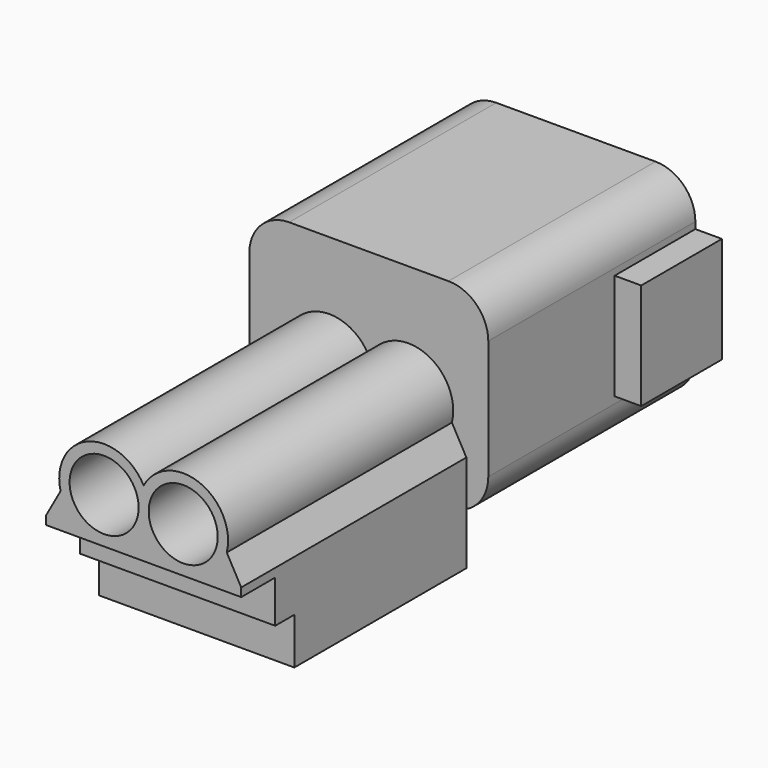
from build123d import *

# Parameters (mm, degrees)
F1_DEPTH     = 21.2
F2_W         = 14.7
F2_H         = 3.2
F3_DEPTH     = 6.7
F4_R         = 2.6
F5_DEPTH     = 10
F6_W         = 18
F6_H         = 15
F7_DEPTH     = 11.9
F9_DEPTH     = 7.6
F10_T1_DEPTH = 34.5
F10_T3_DEPTH = 27
F11_W        = 14.7
F11_H        = 1.8
F12_DEPTH    = 3.5


# Not quite as in the source:
# - a fillet or chamfer that OpenCascade refuses, or shapes differently, is made with other operations: its cross-section is extruded or revolved along the edge and cut away or added


with BuildPart() as f1:
    # F0 (on Front) → F1 (new body)
    with BuildSketch(Plane.XZ):
        with BuildLine():
            Line((-7.35, 0.194197055), (-7.35, -7.15))
            Line((-7.35, -7.15), (7.35, -7.15))
            Line((7.35, -7.15), (7.35, 0.194197055))
            Line((7.35, 0.194197055), (6.2603328375, 2.1552506672))
            ThreePointArc((6.2603328375, 2.1552506672), (3.3980247264, -0.3840505852), (0, 1.375007837))
            ThreePointArc((0, 1.375007837), (-3.3980247264, -0.3840505852), (-6.2603328375, 2.1552506672))
            Line((-6.2603328375, 2.1552506672), (-7.35, 0.194197055))
        make_face()
        with BuildLine():
            ThreePointArc((0, 4.564992163), (-4.1941925187, 6.1243837001), (-6.2603328375, 2.1552506672))
            ThreePointArc((-6.2603328375, 2.1552506672), (-3.3980247264, -0.3840505852), (0, 1.375007837))
            ThreePointArc((0, 1.375007837), (3.3980247264, -0.3840505852), (6.2603328375, 2.1552506672))
            ThreePointArc((6.2603328375, 2.1552506672), (4.1941925187, 6.1243837001), (0, 4.564992163))
        make_face()
    extrude(amount=F1_DEPTH)

    # F2 (on face) → F3 (cut)
    with BuildSketch(Plane(origin=(0, 0, -7.15), x_dir=(1, 0, 0), z_dir=(0, 0, -1))):
        with Locations((0, 19.6)):
            Rectangle(F2_W, F2_H)
    extrude(amount=-F3_DEPTH, mode=Mode.SUBTRACT)

    # F4 (on face) → F5 (cut)
    with BuildSketch(Plane.XZ.offset(21.2)):
        with Locations((-2.98, 2.97)):
            Circle(F4_R)
        with Locations((2.98, 2.97)):
            Circle(F4_R)
    extrude(amount=-F5_DEPTH, mode=Mode.SUBTRACT)

    # F6 (on face) → F7 (join)
    with BuildSketch(Plane(origin=(0, 0, 0), x_dir=(-1, 0, 0), z_dir=(0, 1, 0))):
        with Locations((0, 3.95)):
            Rectangle(F6_W, F6_H)
    extrude(amount=F7_DEPTH)

    # F8 (on face) → F9 (join)
    with BuildSketch(Plane(origin=(0, 11.9, 0), x_dir=(-1, 0, 0), z_dir=(0, 1, 0))):
        Polygon((-9, -0.05), (-9, -3.55), (9, -3.55), (9, -0.05), (11, -0.05), (11, 7.95), (9, 7.95), (9, 11.45), (-9, 11.45), (-9, 7.95), (-11, 7.95), (-11, -0.05), align=None)
    extrude(amount=F9_DEPTH)

    # F10: fillet of radius 3 on 4 edges, made by hand

    # F10_s2 → F10_t1 (cut)
    with BuildSketch(Plane.XZ.offset(-27)):
        with BuildLine():
            ThreePointArc((6, 11.45), (8.1213203436, 10.5713203436), (9, 8.45))
            Line((9, 8.45), (9, 11.45))
            Line((9, 11.45), (6, 11.45))
        make_face()
        with BuildLine():
            ThreePointArc((-9, 8.45), (-8.1213203436, 10.5713203436), (-6, 11.45))
            Line((-6, 11.45), (-9, 11.45))
            Line((-9, 11.45), (-9, 8.45))
        make_face()
    extrude(amount=F10_T1_DEPTH, mode=Mode.SUBTRACT)

    # F10_s4 → F10_t3 (cut)
    with BuildSketch(Plane.XZ.offset(-27)):
        with BuildLine():
            ThreePointArc((6, -3.55), (8.1213203436, -2.6713203436), (9, -0.55))
            Line((9, -0.55), (9, -3.55))
            Line((9, -3.55), (6, -3.55))
        make_face()
        with BuildLine():
            ThreePointArc((-6, -3.55), (-8.1213203436, -2.6713203436), (-9, -0.55))
            Line((-9, -0.55), (-9, -3.55))
            Line((-9, -3.55), (-6, -3.55))
        make_face()
    extrude(amount=F10_T3_DEPTH, mode=Mode.SUBTRACT)

    # F11 (on face) → F12 (cut)
    with BuildSketch(Plane(origin=(0, 0, -7.15), x_dir=(1, 0, 0), z_dir=(0, 0, -1))):
        with Locations((0, 17.1)):
            Rectangle(F11_W, F11_H)
    extrude(amount=-F12_DEPTH, mode=Mode.SUBTRACT)


solid = f1.part
